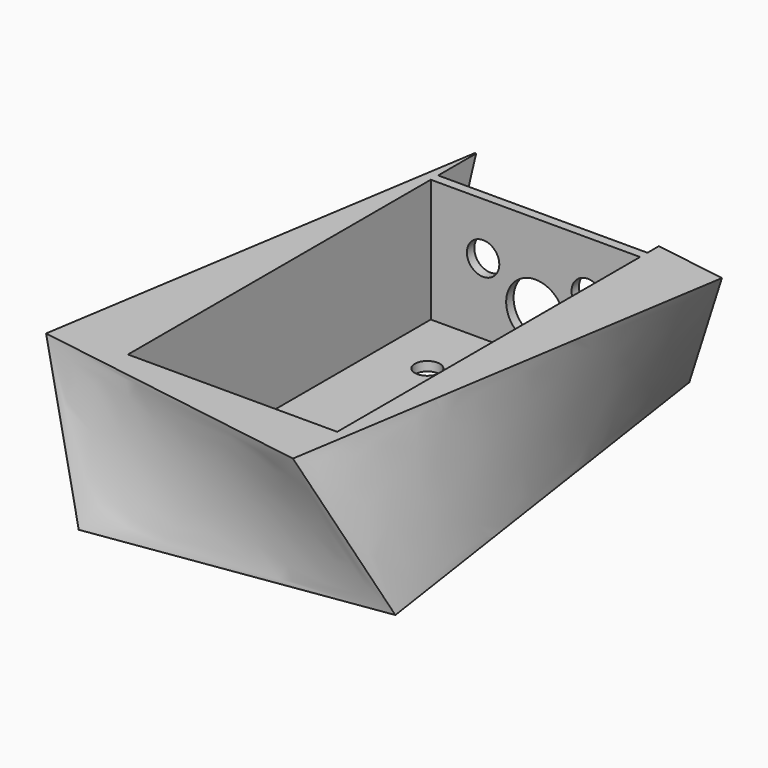
from build123d import *

# Parameters (mm, degrees)
F0_W          = 73
F0_H          = 128
F1_DEPTH      = 43
F5_W          = 68
F5_H          = 123
F6_DEPTH      = 40
F7_R          = 4.071875
F7_R_2        = 6.35
F7_R_3        = 3.675
F8_DEPTH      = 25
F10_R         = 9.5
F10_R_2       = 5.2625
F11_DEPTH     = 15
F12_W         = 68
F12_H         = 40
F13_DEPTH     = 25
F15_TEXT_SIZE = 6.9444444444
F16_DEPTH     = 1.5


# Not quite as in the source:
# - Text() gives the source's letters only with a copy of the font that has no kerning and outlines rounded to 1/6400 em; it was checked with that copy


with BuildPart() as f1:
    # F0 (on Top) → F1 (new body)
    with BuildSketch(Plane.XY):
        Rectangle(F0_W, F0_H)
    extrude(amount=F1_DEPTH)

    # F2 (on face) → F4 section 0
    with BuildSketch(Plane(origin=(0, 0, 0), x_dir=(1, 0, 0), z_dir=(0, 0, -1))):
        Polygon((-56.8218181426, -66.4042994314), (35.1783574532, -80.0045821619), (56.8218181426, 66.4042994314), (-35.1783574532, 80.0045821619), align=None)
    # F3 (on face) → F4 section 1
    with BuildSketch(Plane.XY.offset(43)):
        Polygon((57.4444717884, 65.4410459638), (-34.410543887, 79.9894512126), (-57.4444717884, -65.4410459638), (34.410543887, -79.9894512126), align=None)
    loft()

    # F5 (on face) → F6 (cut)
    with BuildSketch(Plane.XY.offset(43)):
        Rectangle(F5_W, F5_H)
    extrude(amount=-F6_DEPTH, mode=Mode.SUBTRACT)

    # F7 (on face) → F8 (cut)
    with BuildSketch(Plane.XY.offset(3)):
        with Locations((-17.9119046929, 40)):
            Circle(F7_R)
        with Locations((0, 40)):
            Circle(F7_R)
        with Locations((17.9119046929, 40)):
            Circle(F7_R)
        with Locations((0, -33)):
            Circle(F7_R_2)
        with Locations((8.9559523465, 15)):
            Circle(F7_R_3)
        Circle(F7_R_3)
    extrude(amount=-F8_DEPTH, mode=Mode.SUBTRACT)

    # F10 (on offset) → F11 (cut, symmetric)
    with BuildSketch(Plane.XZ.offset(-64.5)):
        with Locations((0, 16)):
            Circle(F10_R)
        with Locations((17, 26)):
            Circle(F10_R_2)
        with Locations((-17, 26)):
            Circle(F10_R_2)
    extrude(amount=F11_DEPTH, both=True, mode=Mode.SUBTRACT)

    # F12 (on offset) → F13 (cut)
    with BuildSketch(Plane.XZ.offset(-64.5)):
        with Locations((0, 23)):
            Rectangle(F12_W, F12_H)
    extrude(amount=-F13_DEPTH, mode=Mode.SUBTRACT)

    # F15 (on face) → F16 (cut)
    with BuildSketch(Plane(origin=(0, 0, 0), x_dir=(1, 0, 0), z_dir=(0, 0, -1))):
        with Locations(Location((29.3945663914, -53), (0, 0, 180))):
            Text('VOL', F15_TEXT_SIZE, font='Open Sans', font_style=FontStyle.BOLD, text_align=(TextAlign.LEFT, TextAlign.BOTTOM))
        with Locations(Location((9.5616319444, -53), (0, 0, 180))):
            Text('TONE', F15_TEXT_SIZE, font='Open Sans', font_style=FontStyle.BOLD, text_align=(TextAlign.LEFT, TextAlign.BOTTOM))
        with Locations(Location((-11.8034205581, -53), (0, 0, 180))):
            Text('GAIN', F15_TEXT_SIZE, font='Open Sans', font_style=FontStyle.BOLD, text_align=(TextAlign.LEFT, TextAlign.BOTTOM))
    extrude(amount=-F16_DEPTH, mode=Mode.SUBTRACT)


solid = f1.part
